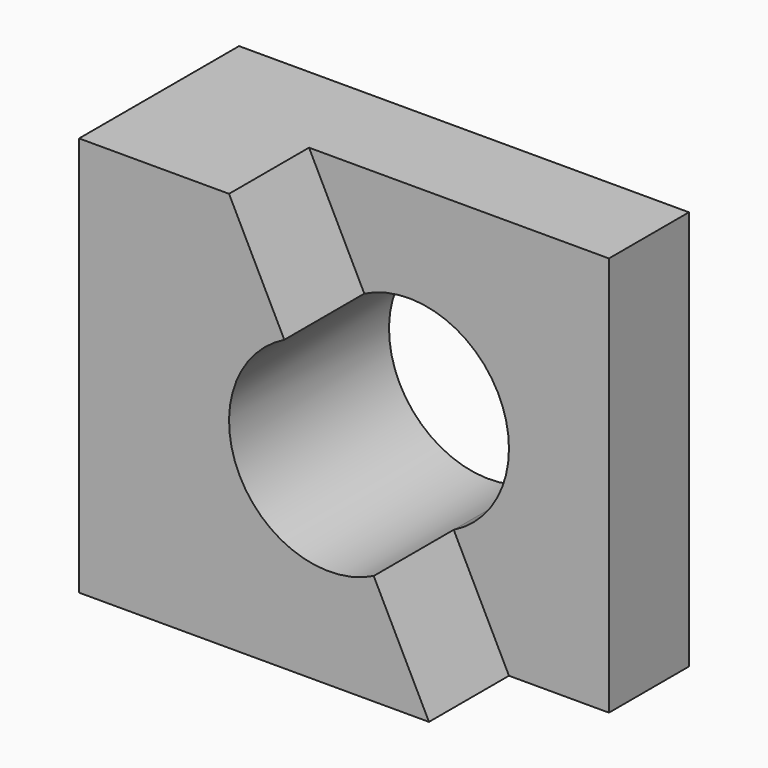
from build123d import *

# Parameters (mm, degrees)
F0_W     = 57.15
F0_H     = 50.8
F1_DEPTH = 25.4
F3_DEPTH = 12.7
F5_DEPTH = 25.4


# Not quite as in the source:
# - a feature of the source that left no trace in its solid (it failed there, or was rolled back) is left out


with BuildPart() as f1:
    # F0 (on Front) → F1 (new body)
    with BuildSketch(Plane.XZ):
        with Locations((28.575, 25.4)):
            Rectangle(F0_W, F0_H)
    extrude(amount=F1_DEPTH)

    # F2 (on face) → F3 (cut)
    with BuildSketch(Plane.XZ.offset(25.4)):
        Polygon((44.45, 0), (57.15, 0), (57.15, 50.8), (19.05, 50.8), align=None)
    extrude(amount=-F3_DEPTH, mode=Mode.SUBTRACT)

    # F4 (on face) → F5 (cut)
    with BuildSketch(Plane.XZ.offset(25.4)):
        with BuildLine():
            ThreePointArc((37.4296126628, 14.0407746743), (42.5532652661, 18.7232148761), (44.45, 25.4))
            ThreePointArc((44.45, 25.4), (38.4267851239, 36.2032652661), (26.0703873372, 36.7592253257))
            Line((26.0703873372, 36.7592253257), (37.4296126628, 14.0407746743))
        make_face()
        with BuildLine():
            Line((37.4296126628, 14.0407746743), (26.0703873372, 36.7592253257))
            ThreePointArc((26.0703873372, 36.7592253257), (20.3907746743, 19.7203873372), (37.4296126628, 14.0407746743))
        make_face()
    extrude(amount=-F5_DEPTH, mode=Mode.SUBTRACT)


solid = f1.part
